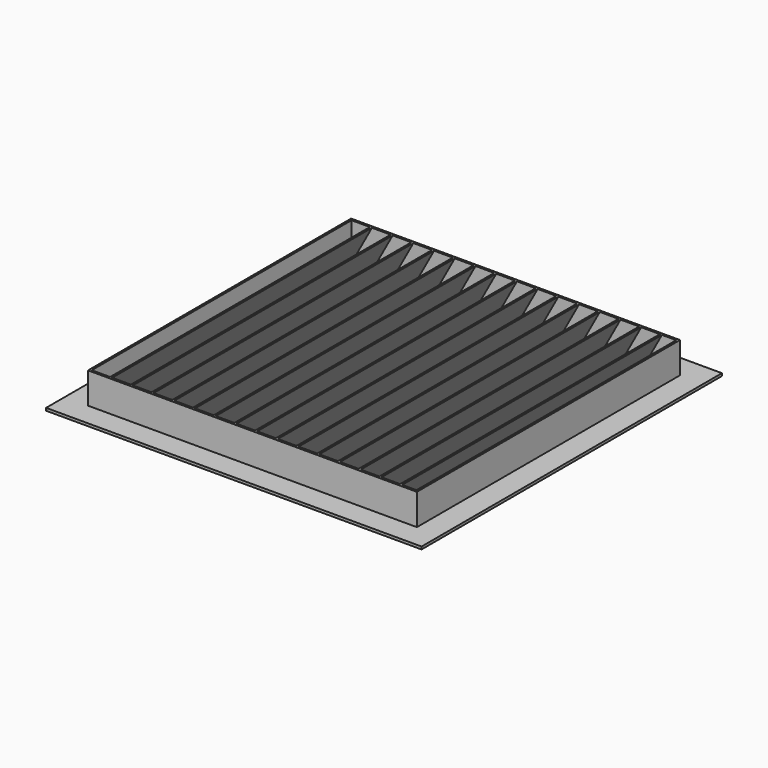
from build123d import *

# Parameters (mm, degrees)
F0_W          = 145
F0_H          = 145
F0_W_2        = 127
F0_H_2        = 127
F0_W_3        = 125.4
F0_H_3        = 125.4
F1_DEPTH      = 1
F2_DEPTH      = 13
F4_DEPTH      = 126
F4_DEPTH_BACK = 0.8


# Not quite as in the source:
# - a feature names something its author has since deleted; it is built from what else it names


with BuildPart() as f1:
    # F0 (on Top) → F1 (new body)
    with BuildSketch(Plane.XY):
        Rectangle(F0_W, F0_H)
        Rectangle(F0_W_2, F0_H_2, mode=Mode.SUBTRACT)
        Rectangle(F0_W_2, F0_H_2)
        Rectangle(F0_W_3, F0_H_3, mode=Mode.SUBTRACT)
    extrude(amount=F1_DEPTH)

    # F0 (on Top) → F2 (join)
    with BuildSketch(Plane.XY):
        Rectangle(F0_W_2, F0_H_2)
        Rectangle(F0_W_3, F0_H_3, mode=Mode.SUBTRACT)
    extrude(amount=F2_DEPTH)


with BuildPart() as f4:
    # F3 (on face) → F4 (new body, two sides)
    with BuildSketch(Plane.XZ.offset(-62.7)) as f4_sk:
        Polygon((-55.6109249592, 13), (-62.7, 0), (-61.9, 0), (-54.8109249592, 13), align=None)
    extrude(amount=F4_DEPTH)
    extrude(f4_sk.sketch, amount=-F4_DEPTH_BACK)


with BuildPart() as f4b:
    # F3 (on face) → F4, piece 2 (new body, two sides)
    with BuildSketch(Plane.XZ.offset(-62.7)) as f4_2_sk:
        Polygon((-47.6109249592, 13), (-54.7, 0), (-53.9, 0), (-46.8109249592, 13), align=None)
    extrude(amount=F4_DEPTH)
    extrude(f4_2_sk.sketch, amount=-F4_DEPTH_BACK)


with BuildPart() as f4c:
    # F3 (on face) → F4, piece 3 (new body, two sides)
    with BuildSketch(Plane.XZ.offset(-62.7)) as f4_3_sk:
        Polygon((-39.6109249592, 13), (-46.7, 0), (-45.9, 0), (-38.8109249592, 13), align=None)
    extrude(amount=F4_DEPTH)
    extrude(f4_3_sk.sketch, amount=-F4_DEPTH_BACK)


with BuildPart() as f4d:
    # F3 (on face) → F4, piece 4 (new body, two sides)
    with BuildSketch(Plane.XZ.offset(-62.7)) as f4_4_sk:
        Polygon((-31.6109249592, 13), (-38.7, 0), (-37.9, 0), (-30.8109249592, 13), align=None)
    extrude(amount=F4_DEPTH)
    extrude(f4_4_sk.sketch, amount=-F4_DEPTH_BACK)


with BuildPart() as f4e:
    # F3 (on face) → F4, piece 5 (new body, two sides)
    with BuildSketch(Plane.XZ.offset(-62.7)) as f4_5_sk:
        Polygon((-23.6109249592, 13), (-30.7, 0), (-29.9, 0), (-22.8109249592, 13), align=None)
    extrude(amount=F4_DEPTH)
    extrude(f4_5_sk.sketch, amount=-F4_DEPTH_BACK)


with BuildPart() as f4f:
    # F3 (on face) → F4, piece 6 (new body, two sides)
    with BuildSketch(Plane.XZ.offset(-62.7)) as f4_6_sk:
        Polygon((-15.6109249592, 13), (-22.7, 0), (-21.9, 0), (-14.8109249592, 13), align=None)
    extrude(amount=F4_DEPTH)
    extrude(f4_6_sk.sketch, amount=-F4_DEPTH_BACK)


with BuildPart() as f4g:
    # F3 (on face) → F4, piece 7 (new body, two sides)
    with BuildSketch(Plane.XZ.offset(-62.7)) as f4_7_sk:
        Polygon((-7.6109249592, 13), (-14.7, 0), (-13.9, 0), (-6.8109249592, 13), align=None)
    extrude(amount=F4_DEPTH)
    extrude(f4_7_sk.sketch, amount=-F4_DEPTH_BACK)


with BuildPart() as f4h:
    # F3 (on face) → F4, piece 8 (new body, two sides)
    with BuildSketch(Plane.XZ.offset(-62.7)) as f4_8_sk:
        Polygon((0.3890750408, 13), (-6.7, 0), (-5.9, 0), (1.1890750408, 13), align=None)
    extrude(amount=F4_DEPTH)
    extrude(f4_8_sk.sketch, amount=-F4_DEPTH_BACK)


with BuildPart() as f4i:
    # F3 (on face) → F4, piece 9 (new body, two sides)
    with BuildSketch(Plane.XZ.offset(-62.7)) as f4_9_sk:
        Polygon((8.3890750408, 13), (1.3, 0), (2.1, 0), (9.1890750408, 13), align=None)
    extrude(amount=F4_DEPTH)
    extrude(f4_9_sk.sketch, amount=-F4_DEPTH_BACK)


with BuildPart() as f4j:
    # F3 (on face) → F4, piece 10 (new body, two sides)
    with BuildSketch(Plane.XZ.offset(-62.7)) as f4_10_sk:
        Polygon((16.3890750408, 13), (9.3, 0), (10.1, 0), (17.1890750408, 13), align=None)
    extrude(amount=F4_DEPTH)
    extrude(f4_10_sk.sketch, amount=-F4_DEPTH_BACK)


with BuildPart() as f4k:
    # F3 (on face) → F4, piece 11 (new body, two sides)
    with BuildSketch(Plane.XZ.offset(-62.7)) as f4_11_sk:
        Polygon((24.3890750408, 13), (17.3, 0), (18.1, 0), (25.1890750408, 13), align=None)
    extrude(amount=F4_DEPTH)
    extrude(f4_11_sk.sketch, amount=-F4_DEPTH_BACK)


with BuildPart() as f4l:
    # F3 (on face) → F4, piece 12 (new body, two sides)
    with BuildSketch(Plane.XZ.offset(-62.7)) as f4_12_sk:
        Polygon((32.3890750408, 13), (25.3, 0), (26.1, 0), (33.1890750408, 13), align=None)
    extrude(amount=F4_DEPTH)
    extrude(f4_12_sk.sketch, amount=-F4_DEPTH_BACK)


with BuildPart() as f4m:
    # F3 (on face) → F4, piece 13 (new body, two sides)
    with BuildSketch(Plane.XZ.offset(-62.7)) as f4_13_sk:
        Polygon((40.3890750408, 13), (33.3, 0), (34.1, 0), (41.1890750408, 13), align=None)
    extrude(amount=F4_DEPTH)
    extrude(f4_13_sk.sketch, amount=-F4_DEPTH_BACK)


with BuildPart() as f4n:
    # F3 (on face) → F4, piece 14 (new body, two sides)
    with BuildSketch(Plane.XZ.offset(-62.7)) as f4_14_sk:
        Polygon((48.3890750408, 13), (41.3, 0), (42.1, 0), (49.1890750408, 13), align=None)
    extrude(amount=F4_DEPTH)
    extrude(f4_14_sk.sketch, amount=-F4_DEPTH_BACK)


with BuildPart() as f4o:
    # F3 (on face) → F4, piece 15 (new body, two sides)
    with BuildSketch(Plane.XZ.offset(-62.7)) as f4_15_sk:
        Polygon((56.3890750408, 13), (49.3, 0), (50.1, 0), (57.1890750408, 13), align=None)
    extrude(amount=F4_DEPTH)
    extrude(f4_15_sk.sketch, amount=-F4_DEPTH_BACK)


solid = Compound([f1.part, f4.part, f4b.part, f4c.part, f4d.part, f4e.part, f4f.part, f4g.part, f4h.part, f4i.part, f4j.part, f4k.part, f4l.part, f4m.part, f4n.part, f4o.part])
